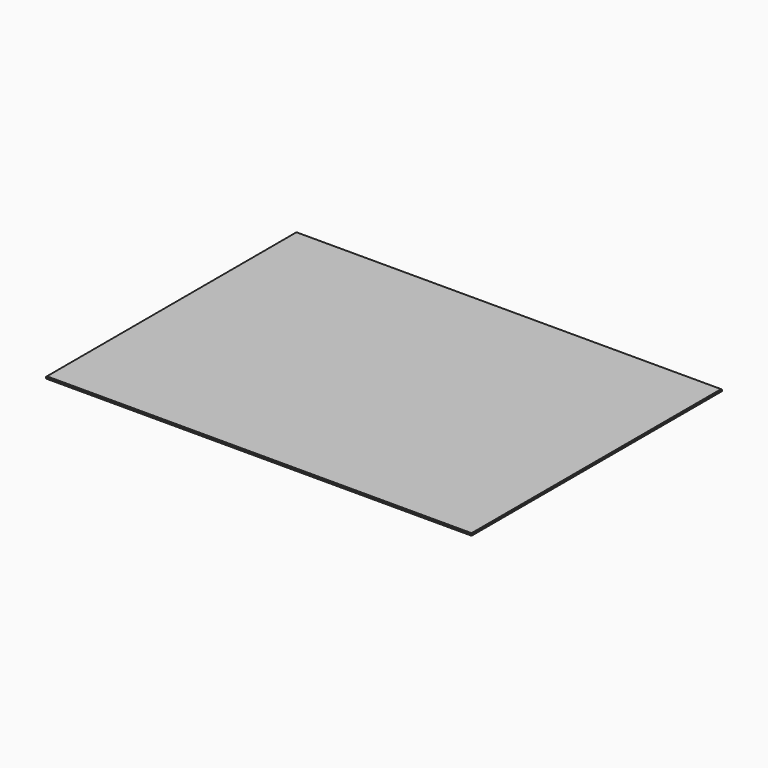
from build123d import *

# Parameters (mm, degrees)
F0_W     = 925
F0_H     = 680
F1_DEPTH = 2.5
F2_SIZE  = 1
F3_SIZE  = 1


with BuildPart() as f1:
    # F0 (on Top) → F1 (new body, symmetric)
    with BuildSketch(Plane.XY):
        Rectangle(F0_W, F0_H)
    extrude(amount=F1_DEPTH, both=True)

    # F2
    f2_edges = [f1.edges().sort_by_distance(p)[0] for p in [
        (0, -340, 2.5),
        (462.5, 0, 2.5),
        (0, 340, 2.5),
        (-462.5, 0, 2.5),
    ]]
    chamfer(f2_edges, length=F2_SIZE)

    # F3
    f3_edges = [f1.edges().sort_by_distance(p)[0] for p in [
        (0, 340, -2.5),
        (462.5, 0, -2.5),
        (0, -340, -2.5),
        (-462.5, 0, -2.5),
    ]]
    chamfer(f3_edges, length=F3_SIZE)


solid = f1.part
